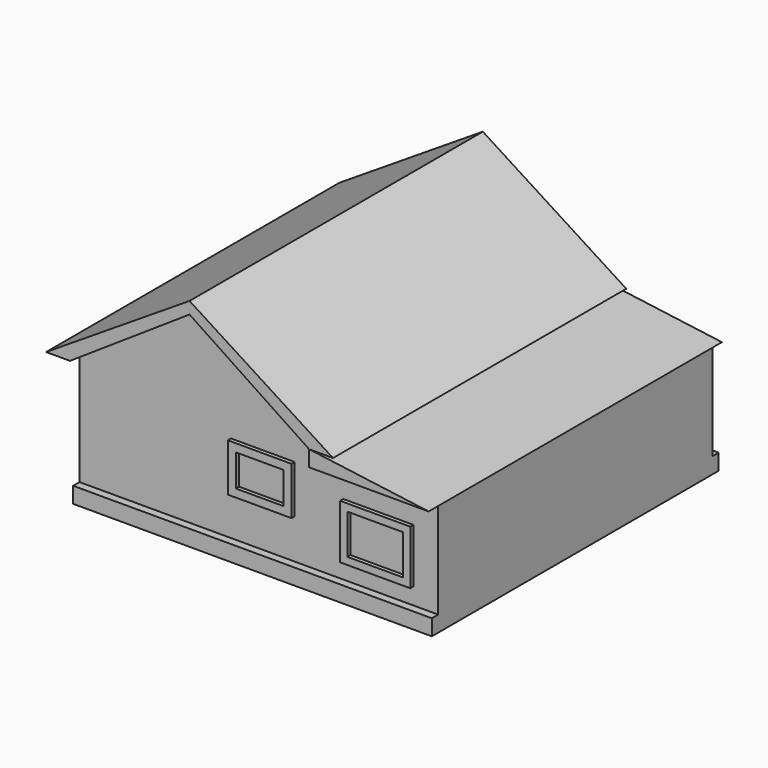
from build123d import *

# Parameters (mm, degrees)
F1_DEPTH     = 7010.4
F2_DEPTH     = 7010.4
F0_W         = 2438.4
F0_H         = 1828.8
F0_W_2       = 4572
F0_H_2       = 3657.6
F0_W_3       = 2682.2400867462
F0_H_3       = 2072.6400867462
F3_DEPTH     = 6553.2
F4_DEPTH     = 6553.2
F0_W_4       = 2133.6
F0_H_4       = 1524
F0_W_5       = 1828.8
F0_H_5       = 1219.2
F5_DEPTH     = 6705.6
F6_DEPTH     = 6553.2
F0_H_6       = 609.6
F7_DEPTH     = 6858
F8_TEXT_SIZE = 1538.9614635044
F9_DEPTH     = 853.44


# Not quite as in the source:
# - Text() gives the source's letters only with a copy of the font that has no kerning and outlines rounded to 1/6400 em; it was checked with that copy


with BuildPart() as f1:
    # F0 (on Front) → F1 (new body, symmetric)
    with BuildSketch(Plane.XZ):
        Polygon((-4577, 0), (-4572, 0), (0, 3048), (0, 3505.2), (-5486.4, 0), align=None)
        Polygon((0, 3048), (4572, 0), (5486.4, 0), (0, 3505.2), align=None)
    extrude(amount=F1_DEPTH, both=True)


with BuildPart() as f2:
    # F0 (on Front) → F2 (new body, symmetric)
    with BuildSketch(Plane.XZ):
        Polygon((9144, -609.6), (4572, 0), (4572, -609.6), align=None)
    extrude(amount=F2_DEPTH, both=True)


with BuildPart() as f3:
    # F0 (on Front) → F3 (new body, symmetric)
    with BuildSketch(Plane.XZ):
        Polygon((-4572, 0), (0, 0), (0, 3048), align=None)
        Polygon((0, 3048), (0, 0), (4572, 0), align=None)
        Polygon((4572, 0), (0, 0), (-4572, 0), (-4572, -4267.2), (-3324.8365304687, -4267.2), (-3352.8, -2133.7832558143), (-2105.6365304687, -2133.6), (-2105.6365304687, -4267.2), (4572, -4267.2), (4572, -609.6), align=None)
        with Locations((2438.4, -1828.8)):
            Rectangle(F0_W, F0_H, mode=Mode.SUBTRACT)
        with Locations((6858, -2438.4)):
            Rectangle(F0_W_2, F0_H_2)
        with Locations((6858, -2590.8)):
            Rectangle(F0_W_3, F0_H_3, mode=Mode.SUBTRACT)
    extrude(amount=F3_DEPTH, both=True)

    # F0 (on Front) → F4 (join, symmetric)
    with BuildSketch(Plane.XZ):
        Polygon((-3352.8, -2133.7832558143), (-3324.8365304687, -4267.2), (-2105.6365304687, -4267.2), (-2105.6365304687, -2133.6), align=None)
    extrude(amount=F4_DEPTH, both=True)

    # F0 (on Front) → F5 (join, symmetric)
    with BuildSketch(Plane.XZ):
        with Locations((6858, -2590.8)):
            Rectangle(F0_W_3, F0_H_3)
        with Locations((6858, -2590.8)):
            Rectangle(F0_W_4, F0_H_4, mode=Mode.SUBTRACT)
        with Locations((2438.4, -1828.8)):
            Rectangle(F0_W, F0_H)
        with Locations((2438.4, -1828.8)):
            Rectangle(F0_W_5, F0_H_5, mode=Mode.SUBTRACT)
    extrude(amount=F5_DEPTH, both=True)

    # F0 (on Front) → F6 (join, symmetric)
    with BuildSketch(Plane.XZ):
        with Locations((2438.4, -1828.8)):
            Rectangle(F0_W_5, F0_H_5)
        with Locations((6858, -2590.8)):
            Rectangle(F0_W_4, F0_H_4)
    extrude(amount=F6_DEPTH, both=True)

    # F0 (on Front) → F7 (join, symmetric)
    with BuildSketch(Plane.XZ):
        Polygon((-3324.8365304687, -4267.2), (-4572, -4267.2), (-4572, -4876.8), (4572, -4876.8), (4572, -4267.2), (-2105.6365304687, -4267.2), align=None)
        with Locations((6858, -4572)):
            Rectangle(F0_W_2, F0_H_6)
    extrude(amount=F7_DEPTH, both=True)


with BuildPart() as f9:
    # F8 (on Front) → F9 (new body)
    with BuildSketch(Plane.XZ):
        with Locations((-3383.0027580261, -6309.1645240784)):
            Text('Trevor Cox', F8_TEXT_SIZE, font='Open Sans', font_style=FontStyle.BOLD, text_align=(TextAlign.LEFT, TextAlign.BOTTOM))
    extrude(amount=F9_DEPTH)


solid = Compound([f1.part, f2.part, f3.part, f9.part])
